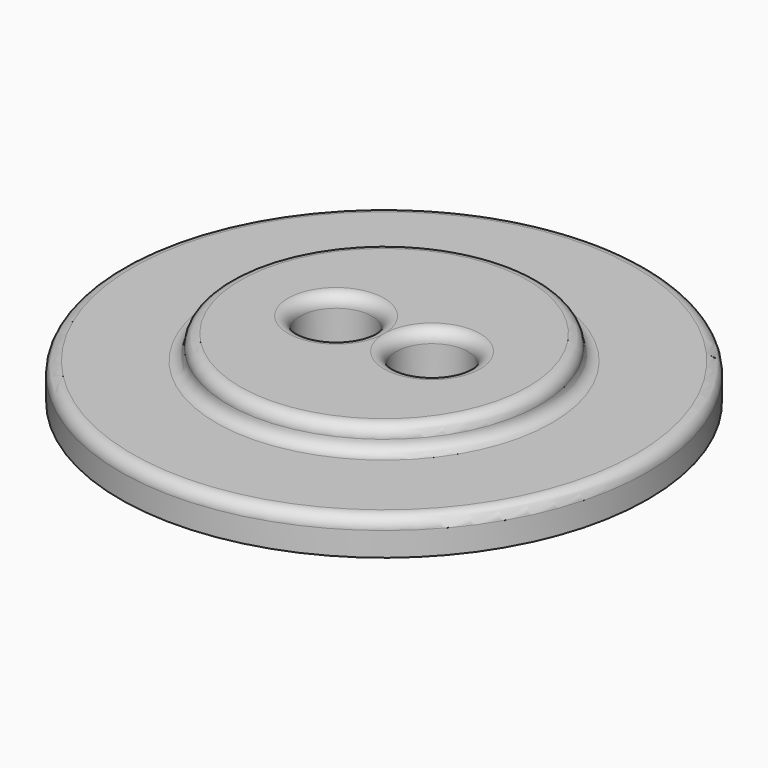
from build123d import *

# Parameters (mm, degrees)
F0_R     = 11
F0_R_2   = 6.5
F1_DEPTH = 1.5
F0_R_3   = 1.5
F2_DEPTH = 2.5
F3_R     = 0.49999


# Not quite as in the source:
# - a fillet or chamfer is up to 0.001 mm smaller than in the source, because OpenCascade refuses the exact size


with BuildPart() as f1:
    # F0 (on Top) → F1 (new body)
    with BuildSketch(Plane.XY):
        Circle(F0_R)
        Circle(F0_R_2, mode=Mode.SUBTRACT)
    extrude(amount=F1_DEPTH)

    # F0 (on Top) → F2 (join)
    with BuildSketch(Plane.XY):
        Circle(F0_R_2)
        with Locations((-2, 0)):
            Circle(F0_R_3, mode=Mode.SUBTRACT)
        with Locations((2, 0)):
            Circle(F0_R_3, mode=Mode.SUBTRACT)
    extrude(amount=F2_DEPTH)

    # F3 (radius 0.5 in the source; OpenCascade refuses exactly that, so slightly less here)
    f3_edges = [f1.edges().sort_by_distance(p)[0] for p in [
        (-11, 0, 1.5),
        (-6.5, 0, 1.5),
        (-6.5, 0, 2.5),
        (0.5, 0, 2.5),
        (-3.5, 0, 2.5),
    ]]
    fillet(f3_edges, radius=F3_R)


solid = f1.part
